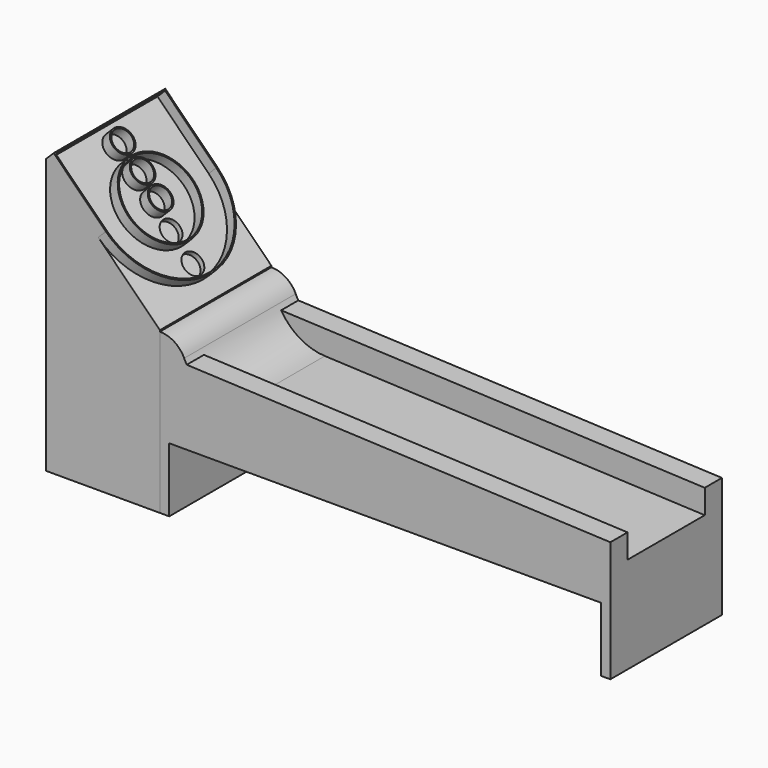
from build123d import *

# Parameters (mm, degrees)
F2_DEPTH  = 330.2
F4_DEPTH  = 330.2
F5_R      = 190.5
F5_R_2    = 184.15
F5_R_3    = 57.15
F5_R_4    = 50.8
F6_DEPTH  = 50.8
F7_DEPTH  = 25.4
F9_DEPTH  = 101.6
F11_DEPTH = 101.6


# Not quite as in the source:
# - a variable given as a bare number and used for a length is read in inches; the dataset says mm whatever the document's units were


with BuildPart() as f2:
    # F1 (on Front) → F2 (new body, symmetric)
    with BuildSketch(Plane.XZ):
        with BuildLine():
            Line((-44.45, 0), (0, 0))
            Line((0, 0), (0, 457.2))
            Line((0, 457.2), (-1799.1673024383, 535.7533408746))
            ThreePointArc((-1799.1673024383, 535.7533408746), (-1929.3267001402, 578.3588586439), (-2018.4989110463, 682.306036367))
            ThreePointArc((-2018.4989110463, 682.306036367), (-2065.36294974, 735.7442307441), (-2133.6, 755.6335171259))
            Line((-2133.6, 755.6335171259), (-2133.6, 0))
            Line((-2133.6, 0), (-2089.15, 0))
            Line((-2089.15, 0), (-2089.15, 304.8))
            Line((-2089.15, 304.8), (-44.45, 304.8))
            Line((-44.45, 304.8), (-44.45, 0))
        make_face()
    extrude(amount=F2_DEPTH, both=True)

    # F8 (on face) → F9 (join)
    with BuildSketch(Plane.XZ.offset(330.2)):
        with BuildLine():
            Line((-1799.1673024383, 535.7533408746), (0, 457.2))
            Line((0, 457.2), (0, 571.5))
            Line((0, 571.5), (-2006.1747965862, 659.0914832582))
            ThreePointArc((-2006.1747965862, 659.0914832582), (-1918.2110987992, 571.3404020762), (-1799.1673024383, 535.7533408746))
        make_face()
    extrude(amount=-F9_DEPTH)

    # F10 (on face) → F11 (join)
    with BuildSketch(Plane(origin=(0, 330.2, 0), x_dir=(-1, 0, 0), z_dir=(0, 1, 0))):
        with BuildLine():
            Line((2006.1747965862, 659.0914832582), (0, 571.5))
            Line((0, 571.5), (0, 457.2))
            Line((0, 457.2), (1799.1673024383, 535.7533408746))
            ThreePointArc((1799.1673024383, 535.7533408746), (1918.2110987992, 571.3404020762), (2006.1747965862, 659.0914832582))
        make_face()
    extrude(amount=-F11_DEPTH)


with BuildPart() as f4:
    # F3 (on Front) → F4 (new body, symmetric)
    with BuildSketch(Plane.XZ):
        Polygon((-2672.4153672641, 0), (-2133.6, 0), (-2133.6, 762), (-2672.4153672641, 1300.8153672641), align=None)
    extrude(amount=F4_DEPTH, both=True)

    # F5 (on face) → F6 (join)
    with BuildSketch(Plane(origin=(-685.8, 0, -685.8), x_dir=(0.7071067812, 0, -0.7071067812), z_dir=(0.7071067812, 0, 0.7071067812))):
        with BuildLine():
            Line((-2809.4983956038, -330.2), (-2460.2483956038, -330.2))
            ThreePointArc((-2460.2483956038, -330.2), (-2130.0483956038, 0), (-2460.2483956038, 330.2))
            Line((-2460.2483956038, 330.2), (-2809.4983956038, 330.2))
            Line((-2809.4983956038, 330.2), (-2809.4983956038, -330.2))
        make_face()
        with BuildLine():
            ThreePointArc((-2460.2483956038, 323.85), (-2136.3983956038, 0), (-2460.2483956038, -323.85))
            Line((-2460.2483956038, -323.85), (-2803.1483956038, -323.85))
            Line((-2803.1483956038, -323.85), (-2803.1483956038, 323.85))
            Line((-2803.1483956038, 323.85), (-2460.2483956038, 323.85))
        make_face(mode=Mode.SUBTRACT)
        with Locations((-2466.5983956038, 0)):
            Circle(F5_R)
        with Locations((-2466.5983956038, 0)):
            Circle(F5_R_2, mode=Mode.SUBTRACT)
        with Locations((-2466.5983956038, 0)):
            Circle(F5_R_3)
        with Locations((-2466.5983956038, 0)):
            Circle(F5_R_4, mode=Mode.SUBTRACT)
        with Locations((-2587.2483956038, 0)):
            Circle(F5_R_3)
        with Locations((-2587.2483956038, 0)):
            Circle(F5_R_4, mode=Mode.SUBTRACT)
        with Locations((-2720.5983956038, 0)):
            Circle(F5_R_3)
        with Locations((-2720.5983956038, 0)):
            Circle(F5_R_4, mode=Mode.SUBTRACT)
    extrude(amount=F6_DEPTH)

    # F5 (on face) → F7 (cut)
    with BuildSketch(Plane(origin=(-685.8, 0, -685.8), x_dir=(0.7071067812, 0, -0.7071067812), z_dir=(0.7071067812, 0, 0.7071067812))):
        with Locations((-2199.8983956038, 0)):
            Circle(F5_R_4)
        with Locations((-2345.9483956038, 0)):
            Circle(F5_R_4)
    extrude(amount=-F7_DEPTH, mode=Mode.SUBTRACT)


solid = Compound([f2.part, f4.part])
